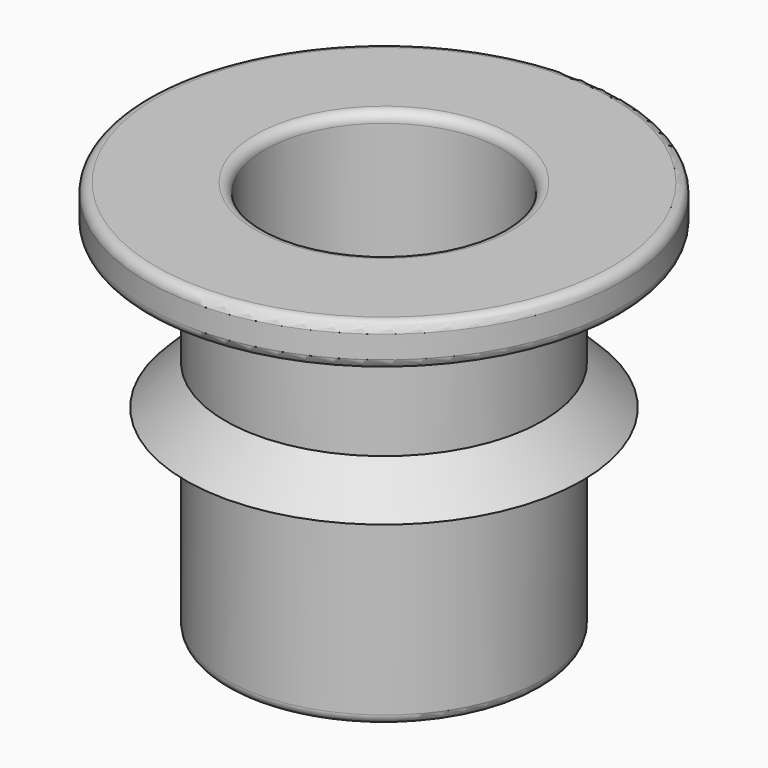
from build123d import *

# Parameters (mm, degrees)
F0_R     = 8
F0_R_2   = 6
F1_DEPTH = 10
F2_R     = 10
F2_R_2   = 6
F3_DEPTH = 2
F4_R     = 8
F4_R_2   = 6
F5_DEPTH = 5
F6_R     = 12
F6_R_2   = 6
F7_DEPTH = 3
F8_SIZE  = 1.99999
F9_SIZE2 = 3
F9_SIZE  = 1


# Not quite as in the source:
# - a fillet or chamfer that OpenCascade refuses, or shapes differently, is made with other operations: its cross-section is extruded or revolved along the edge and cut away or added
# - a fillet or chamfer is up to 0.001 mm smaller than in the source, because OpenCascade refuses the exact size


with BuildPart() as f1:
    # F0 (on Top) → F1 (new body)
    with BuildSketch(Plane.XY):
        Circle(F0_R)
        Circle(F0_R_2, mode=Mode.SUBTRACT)
    extrude(amount=-F1_DEPTH)

    # F2 (on Top) → F3 (join)
    with BuildSketch(Plane.XY):
        Circle(F2_R)
        Circle(F2_R_2, mode=Mode.SUBTRACT)
    extrude(amount=F3_DEPTH)

    # F4 (on face) → F5 (join)
    with BuildSketch(Plane.XY.offset(2)):
        Circle(F4_R)
        Circle(F4_R_2, mode=Mode.SUBTRACT)
    extrude(amount=F5_DEPTH)

    # F6 (on face) → F7 (join)
    with BuildSketch(Plane.XY.offset(7)):
        Circle(F6_R)
        Circle(F6_R_2, mode=Mode.SUBTRACT)
    extrude(amount=F7_DEPTH)

    # F8 (size 2 in the source; OpenCascade refuses exactly that, so slightly less here)
    f8_edges = [f1.edges().sort_by_distance(p)[0] for p in [
        (-10, 0, 2),
    ]]
    chamfer(f8_edges, length=F8_SIZE)

    # F9
    f9_edges = [f1.edges().sort_by_distance(p)[0] for p in [
        (-12, 0, 7),
    ]]
    f9_side = f1.faces().sort_by_distance((-12, 0, 8.5))[0]
    chamfer(f9_edges, length=F9_SIZE, length2=F9_SIZE2, reference=f9_side)

    # F10: fillet of radius 0.5 on 13 edges, made by hand

    # F10_s1 → F10_t2 (revolve, cut)
    with BuildSketch(Plane.XZ):
        with BuildLine():
            ThreePointArc((11.658113883, 7.886037961), (11.9056210926, 8.0680244677), (12, 8.36037961))
            Line((12, 8.36037961), (12, 8))
            Line((12, 8), (11.658113883, 7.886037961))
        make_face()
    revolve(axis=Axis((0, 0, 8), (0, 0, 1)), mode=Mode.SUBTRACT)

    # F10_s3 → F10_t4 (revolve, cut)
    with BuildSketch(Plane.XZ):
        with BuildLine():
            ThreePointArc((12, 9.5), (11.8535533906, 9.8535533906), (11.5, 10))
            Line((11.5, 10), (12, 10))
            Line((12, 10), (12, 9.5))
        make_face()
    revolve(axis=Axis((0, 0, 10), (0, 0, 1)), mode=Mode.SUBTRACT)

    # F10_s5 → F10_t6 (revolve, cut)
    with BuildSketch(Plane.XZ):
        with BuildLine():
            ThreePointArc((6, -9.5), (6.1464466094, -9.8535533906), (6.5, -10))
            Line((6.5, -10), (6, -10))
            Line((6, -10), (6, -9.5))
        make_face()
    revolve(axis=Axis((0, 0, -10), (0, 0, 1)), mode=Mode.SUBTRACT)

    # F10_s7 → F10_t8 (revolve, cut)
    with BuildSketch(Plane.XZ):
        with BuildLine():
            ThreePointArc((6.5, 10), (6.1464466094, 9.8535533906), (6, 9.5))
            Line((6, 9.5), (6, 10))
            Line((6, 10), (6.5, 10))
        make_face()
    revolve(axis=Axis((0, 0, 10), (0, 0, 1)), mode=Mode.SUBTRACT)

    # F10_s9 → F10_t10 (revolve, cut)
    with BuildSketch(Plane.XZ):
        with BuildLine():
            ThreePointArc((8, -9.5), (7.8535533906, -9.8535533906), (7.5, -10))
            Line((7.5, -10), (8, -10))
            Line((8, -10), (8, -9.5))
        make_face()
    revolve(axis=Axis((0, 0, -10), (0, 0, 1)), mode=Mode.SUBTRACT)


solid = f1.part
